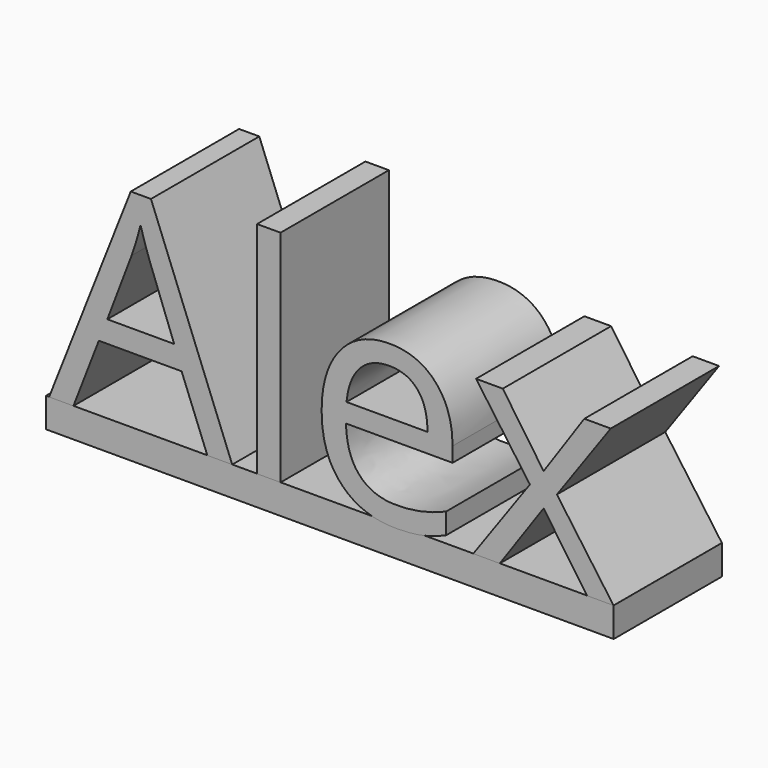
from build123d import *

# Parameters (mm, degrees)
F0_TEXT_SIZE = 34.7334995038
F1_DEPTH     = 16.256
F2_W         = 68.139269948
F2_H         = 16.237936914
F3_DEPTH     = 3.556


# Not quite as in the source:
# - Text() gives the source's letters only with a copy of the font that has no kerning and outlines rounded to 1/6400 em; it was checked with that copy


with BuildPart() as f1:
    # F0 (on Front) → F1 (new body)
    with BuildSketch(Plane.XZ):
        with Locations((-34.5643758774, 0)):
            Text('Alex', F0_TEXT_SIZE, font='Open Sans', text_align=(TextAlign.LEFT, TextAlign.BOTTOM))
    extrude(amount=F1_DEPTH)


with BuildPart() as f3:
    # F2 (on Top) → F3 (new body)
    with BuildSketch(Plane.XY):
        with Locations((-0.8719153702, -8.118968457)):
            Rectangle(F2_W, F2_H)
    extrude(amount=-F3_DEPTH)


solid = Compound([f1.part, f3.part])
